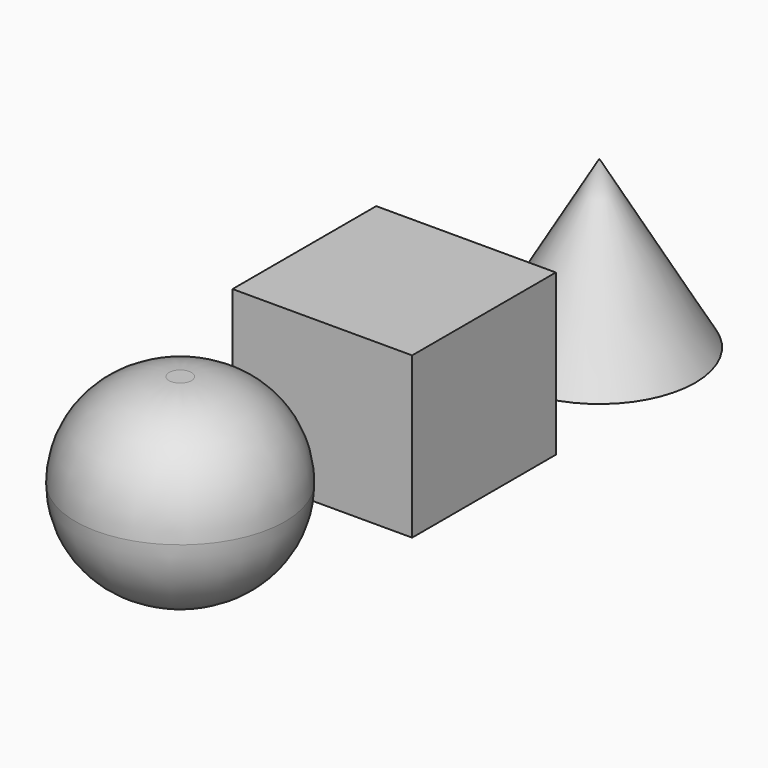
from build123d import *

# Parameters (mm, degrees)
F0_R     = 63.7495375214
F1_DEPTH = 153.67
F1_TAPER = 30
F2_W     = 119.3985827267
F2_H     = 119.398586452
F3_DEPTH = 106.68
F4_R     = 69.6534055832
F5_DEPTH = 124.46
F6_R     = 62.22999


# Not quite as in the source:
# - a fillet or chamfer is up to 0.001 mm smaller than in the source, because OpenCascade refuses the exact size


with BuildPart() as f1:
    # F0 (on Top) → F1 (new body)
    with BuildSketch(Plane.XY):
        Circle(F0_R)
    extrude(amount=F1_DEPTH, taper=F1_TAPER)


with BuildPart() as f3:
    # F2 (on Top) → F3 (new body)
    with BuildSketch(Plane.XY):
        with Locations((-1.9145961851, -168.0913157761)):
            Rectangle(F2_W, F2_H)
    extrude(amount=F3_DEPTH)


with BuildPart() as f5:
    # F4 (on Top) → F5 (new body)
    with BuildSketch(Plane.XY):
        with Locations((0, -348.2365608215)):
            Circle(F4_R)
    extrude(amount=F5_DEPTH)

    # F6 (radius 62.23 in the source; OpenCascade refuses exactly that, so slightly less here)
    f6_edges = [f5.edges().sort_by_distance(p)[0] for p in [
        (-69.653406, -348.236561, 0),
        (-69.653406, -348.236561, 124.46),
    ]]
    fillet(f6_edges, radius=F6_R)


solid = Compound([f1.part, f3.part, f5.part])
